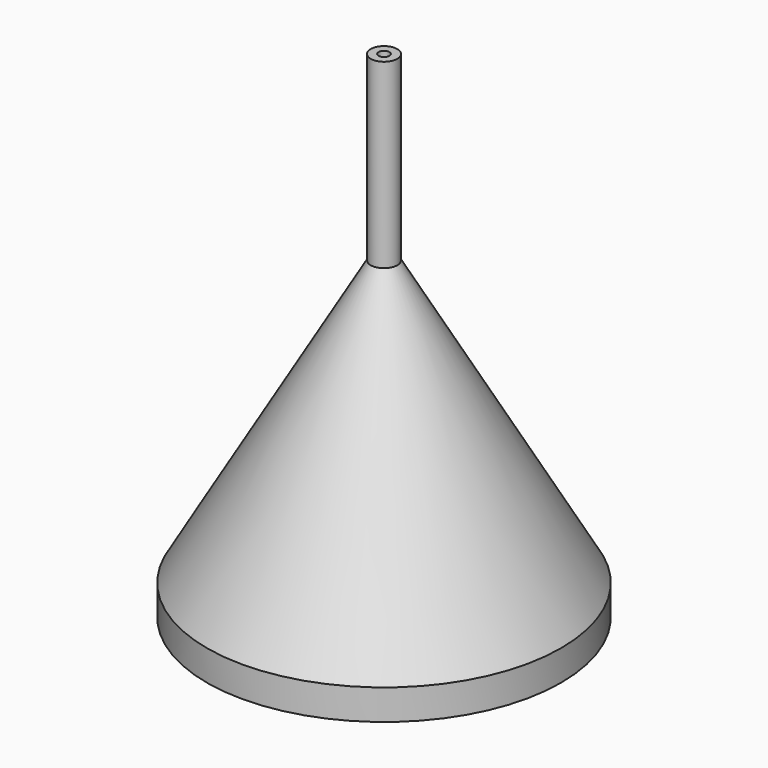
from build123d import *

# Parameters (mm, degrees)
F0_R        = 12.7
F1_DEPTH    = 22.86
F2_R        = 0.9525
F3_DEPTH    = 12.7
F4_R        = 0.381
F5_DEPTH    = 35.561
F6_S5_R     = 0.9525
F6_T6_DEPTH = 22
F7_R        = 11.43
F8_DEPTH    = 1.27
F9_S5_R     = 11.43
F9_T6_DEPTH = 20


# Not quite as in the source:
# - a fillet or chamfer that OpenCascade refuses, or shapes differently, is made with other operations: its cross-section is extruded or revolved along the edge and cut away or added


with BuildPart() as f1:
    # F0 (on Top) → F1 (new body)
    with BuildSketch(Plane.XY):
        with Locations((-32.7860526741, 35.493157804)):
            Circle(F0_R)
    extrude(amount=F1_DEPTH)

    # F2 (on face) → F3 (join)
    with BuildSketch(Plane.XY.offset(22.86)):
        with Locations((-32.7860526741, 35.493157804)):
            Circle(F2_R)
    extrude(amount=F3_DEPTH)

    # F4 (on face) → F5 (cut, through all)
    with BuildSketch(Plane.XY.offset(35.56)):
        with Locations((-32.7860526741, 35.493157804)):
            Circle(F4_R)
    extrude(amount=-F5_DEPTH, mode=Mode.SUBTRACT)

    # F6: chamfer of 11.938 x 20.6772225408 on 1 edges, made by hand


with BuildPart() as f6_tool2:
    # F6_s3 → F6_t4 (revolve)
    with BuildSketch(Plane.XZ.offset(-35.493157804)):
        Polygon((-20.0860526741, 2.1827774592), (-32.0240526741, 22.86), (-20.0860526741, 22.86), align=None)
    revolve(axis=Axis((-32.7860526741, 35.493157804, 22.86), (0, 0, 1)))

    # F6_s5 → F6_t6 (cut, symmetric)
    with BuildSketch(Plane.XY.offset(12.5)):
        with Locations((-32.7860526741, 35.493157804)):
            Circle(F6_S5_R)
    extrude(amount=F6_T6_DEPTH, both=True, mode=Mode.SUBTRACT)


with BuildPart() as f1_1:
    add(f1.part)

    # F6_t1: cut F6_tool2
    add(f6_tool2.part, mode=Mode.SUBTRACT)

    # F7 (on face) → F8 (cut)
    with BuildSketch(Plane(origin=(0, 0, 0), x_dir=(1, 0, 0), z_dir=(0, 0, -1))):
        with Locations((-32.7860526741, -35.493157804)):
            Circle(F7_R)
    extrude(amount=-F8_DEPTH, mode=Mode.SUBTRACT)

    # F9: chamfer of 11.938 on 1 edges, made by hand


with BuildPart() as f9_tool2:
    # F9_s3 → F9_t4 (revolve)
    with BuildSketch(Plane.XZ.offset(-35.493157804)):
        Polygon((-20.4670526741, 1.27), (-32.4050526741, 13.208), (-32.4050526741, 1.27), align=None)
    revolve(axis=Axis((-32.7860526741, 35.493157804, 1.27), (0, 0, 1)))

    # F9_s5 → F9_t6 (intersect, symmetric)
    with BuildSketch(Plane.XY.offset(7.2)):
        with Locations((-32.7860526741, 35.493157804)):
            Circle(F9_S5_R)
    extrude(amount=F9_T6_DEPTH, both=True, mode=Mode.INTERSECT)


with BuildPart() as f1_2:
    add(f1_1.part)

    # F9_t1: cut F9_tool2
    add(f9_tool2.part, mode=Mode.SUBTRACT)


solid = f1_2.part
